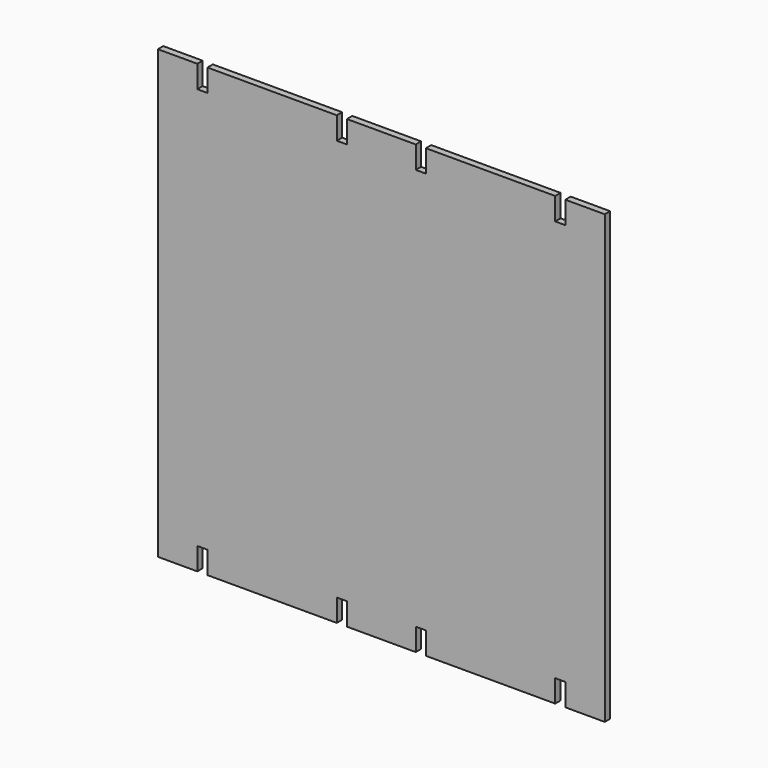
from build123d import *

# Parameters (mm, degrees)
F1_DEPTH = 12


# Not quite as in the source:
# - a feature names something its author has since deleted; it is built from what else it names


with BuildPart() as f1:
    # F0 (on Front) → F1 (new body)
    with BuildSketch(Plane.XZ):
        Polygon((0, 798), (0, 0), (70.5, 0), (70.5, 40), (88.5, 40), (88.5, 0), (319.5, 0), (319.5, 40), (337.5, 40), (337.5, 0), (460.5, 0), (460.5, 40), (478.5, 40), (478.5, 0), (709.5, 0), (709.5, 40), (727.5, 40), (727.5, 0), (798, 0), (798, 798), (727.5, 798), (727.5, 758), (709.5, 758), (709.5, 798), (478.5, 798), (478.5, 758), (460.5, 758), (460.5, 798), (337.5, 798), (337.5, 758), (319.5, 758), (319.5, 798), (88.5, 798), (88.5, 758), (70.5, 758), (70.5, 798), align=None)
    extrude(amount=F1_DEPTH)


solid = f1.part
